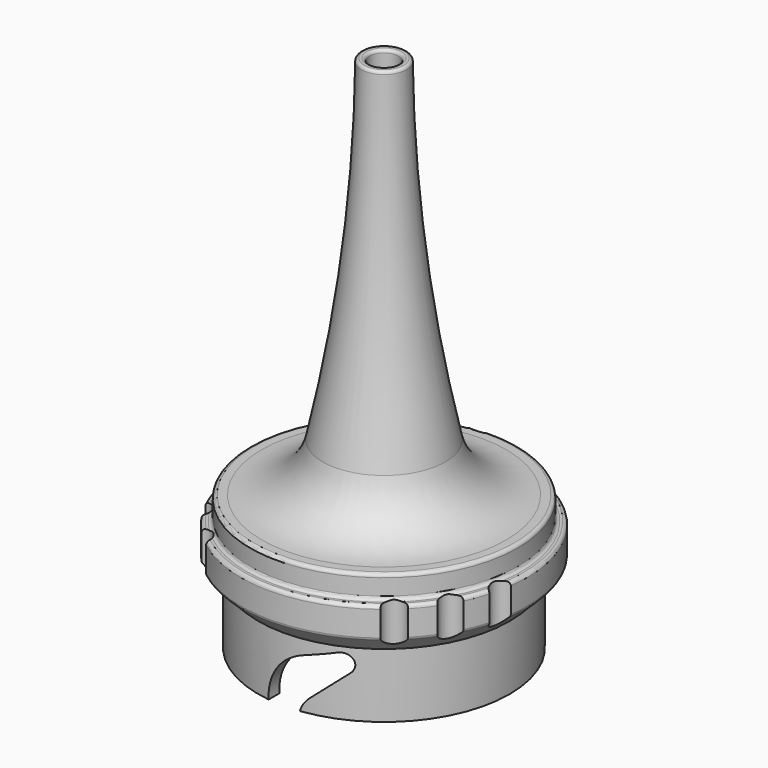
from build123d import *

# Parameters (mm, degrees)
F3_R     = 0.3
F4_R     = 0.25
F5_R     = 1
F6_DEPTH = 25
F8_DEPTH = 25


with BuildPart() as f2:
    # F0 (on Front) → F2 (revolve)
    with BuildSketch(Plane.XZ):
        with BuildLine():
            ThreePointArc((-5.3094973706, 15.8997916811), (-7.2132406442, 12.8574387606), (-10.6, 11.67))
            Line((-10.6, 11.67), (-11.6, 11.67))
            Line((-11.6, 11.67), (-11.6, 9.67))
            Line((-11.6, 9.67), (-12.4, 9.67))
            Line((-12.4, 9.67), (-12.4, 7.07))
            Line((-12.4, 7.07), (-10.9, 5.57))
            Line((-10.9, 5.57), (-10.9, 0))
            Line((-10.9, 0), (-9.75, 0))
            Line((-9.75, 0), (-9.75, 9.6729332581))
            ThreePointArc((-9.75, 9.6729332581), (-5.9481273524, 12.3099372614), (-3.9219260792, 16.4695687526))
            ThreePointArc((-3.9219260792, 16.4695687526), (-1.8409403996, 30.6650116693), (-1.25, 45))
            Line((-1.25, 45), (-1.95, 45))
            ThreePointArc((-1.95, 45), (-2.8507255203, 30.3599608736), (-5.3094973706, 15.8997916811))
        make_face()
    revolve(axis=Axis((0, 0, 0), (0, 0, 1)))

    # F3
    f3_edges = [f2.edges().sort_by_distance(p)[0] for p in [
        (12.4, 0, 9.67),
        (12.4, 0, 7.07),
        (11.6, 0, 11.67),
        (11.6, 0, 9.67),
    ]]
    fillet(f3_edges, radius=F3_R)

    # F4
    f4_edges = [f2.edges().sort_by_distance(p)[0] for p in [
        (1.25, 0, 45),
        (1.95, 0, 45),
    ]]
    fillet(f4_edges, radius=F4_R)

    # F5 (on Top) → F6 (cut)
    with BuildSketch(Plane.XY):
        with Locations((0, 12.7)):
            Circle(F5_R)
        with Locations((-3.9500885061, 12.0700787402)):
            Circle(F5_R)
        with Locations((3.9500885061, 12.0700787402)):
            Circle(F5_R)
        with Locations((-8.4779505616, -9.4559163636)):
            Circle(F5_R)
        with Locations((-10.9985226281, -6.35)):
            Circle(F5_R)
        with Locations((-12.4280390677, -2.6141623766)):
            Circle(F5_R)
        with Locations((12.4280390677, -2.6141623766)):
            Circle(F5_R)
        with Locations((10.9985226281, -6.35)):
            Circle(F5_R)
        with Locations((8.4779505616, -9.4559163636)):
            Circle(F5_R)
    extrude(amount=F6_DEPTH, mode=Mode.SUBTRACT)

    # F7 (on Front) → F8 (cut)
    with BuildSketch(Plane.XZ):
        with BuildLine():
            ThreePointArc((1.7392033478, 4.3713967316), (-0.5625172838, 2.7207434698), (-1.35, 0))
            Line((-1.35, 0), (1.35, 0))
            ThreePointArc((1.35, 0), (1.6498014262, 0.6449388172), (2.1149230126, 1.1829805283))
            Line((2.1149230126, 1.1829805283), (4.8935270099, 3.6156385314))
            ThreePointArc((4.8935270099, 3.6156385314), (5.0779713655, 4.6655839342), (4.091638402, 5.07))
            Line((4.091638402, 5.07), (1.7392033478, 4.3713967316))
        make_face()
    extrude(amount=F8_DEPTH, mode=Mode.SUBTRACT)


solid = f2.part
